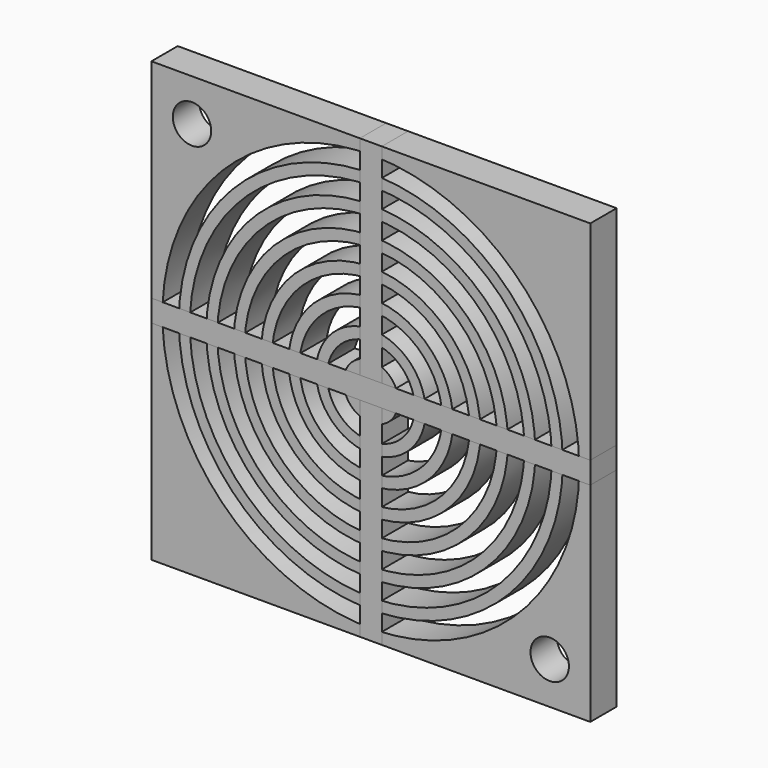
from build123d import *

# Parameters (mm, degrees)
F0_W      = 40
F0_H      = 40
F0_R      = 19
F1_DEPTH  = 3
F2_R      = 1.75
F3_DEPTH  = 5
F6_COUNT  = 2
F8_R      = 10
F8_R_2    = 9
F18_DEPTH = 3
F9_R      = 5
F9_R_2    = 4
F10_R     = 7.5
F10_R_2   = 6.5
F11_R     = 2.5
F11_R_2   = 1.5
F12_R     = 2.5
F13_R     = 12.5
F13_R_2   = 11.5
F14_R     = 15
F14_R_2   = 14
F15_R     = 17.5
F15_R_2   = 16.5
F16_W     = 2
F16_H     = 40
F17_W     = 40
F17_H     = 2


# Not quite as in the source:
# - a feature names something its author has since deleted; it is built from what else it names


with BuildPart() as f1:
    # F0 (on Front) → F1 (new body)
    with BuildSketch(Plane.XZ):
        Rectangle(F0_W, F0_H)
        Circle(F0_R, mode=Mode.SUBTRACT)
    extrude(amount=F1_DEPTH)


with BuildPart() as f3:
    # F2 (on face) → F3 (new body)
    with BuildSketch(Plane(origin=(0, 0, 0), x_dir=(-1, 0, 0), z_dir=(0, 1, 0))):
        with Locations((16.3023483751, 16.1759720192)):
            Circle(F2_R)
    extrude(amount=-F3_DEPTH)


with BuildPart() as f6_1:
    # F6: instance of F3
    add(f3.part.rotate(Axis((0, -5.2183736116, 0), (0, -1, 0)), 1 * 360 / F6_COUNT))


with BuildPart() as f1_1:
    add(f1.part)

    # F7: cut F6_1, F3
    add(f6_1.part, mode=Mode.SUBTRACT)
    add(f3.part, mode=Mode.SUBTRACT)


with BuildPart() as f18:
    # F8 (on face) → F18 (new body)
    with BuildSketch(Plane.XZ.offset(3)):
        Circle(F8_R)
        Circle(F8_R_2, mode=Mode.SUBTRACT)
    extrude(amount=-F18_DEPTH)


with BuildPart() as f18b:
    # F9 (on face) → F18, piece 2 (new body)
    with BuildSketch(Plane.XZ.offset(3)):
        Circle(F9_R)
        Circle(F9_R_2, mode=Mode.SUBTRACT)
    extrude(amount=-F18_DEPTH)


with BuildPart() as f18c:
    # F10 (on face) → F18, piece 3 (new body)
    with BuildSketch(Plane.XZ.offset(3)):
        Circle(F10_R)
        Circle(F10_R_2, mode=Mode.SUBTRACT)
    extrude(amount=-F18_DEPTH)


with BuildPart() as f18d:
    # F11 (on face) → F18, piece 4 (new body)
    with BuildSketch(Plane.XZ.offset(3)):
        Circle(F11_R)
        Circle(F11_R_2, mode=Mode.SUBTRACT)
    extrude(amount=-F18_DEPTH)


with BuildPart() as f18e:
    # F12 (on face) → F18, piece 5 (new body)
    with BuildSketch(Plane.XZ.offset(3)):
        Circle(F12_R)
    extrude(amount=-F18_DEPTH)


with BuildPart() as f18f:
    # F13 (on face) → F18, piece 6 (new body)
    with BuildSketch(Plane.XZ.offset(3)):
        Circle(F13_R)
        Circle(F13_R_2, mode=Mode.SUBTRACT)
    extrude(amount=-F18_DEPTH)


with BuildPart() as f18g:
    # F14 (on face) → F18, piece 7 (new body)
    with BuildSketch(Plane.XZ.offset(3)):
        Circle(F14_R)
        Circle(F14_R_2, mode=Mode.SUBTRACT)
    extrude(amount=-F18_DEPTH)


with BuildPart() as f18h:
    # F15 (on face) → F18, piece 8 (new body)
    with BuildSketch(Plane.XZ.offset(3)):
        Circle(F15_R)
        Circle(F15_R_2, mode=Mode.SUBTRACT)
    extrude(amount=-F18_DEPTH)


with BuildPart() as f18i:
    # F16 (on face) → F18, piece 9 (new body)
    with BuildSketch(Plane.XZ.offset(3)):
        Rectangle(F16_W, F16_H)
    extrude(amount=-F18_DEPTH)


with BuildPart() as f18j:
    # F17 (on face) → F18, piece 10 (new body)
    with BuildSketch(Plane.XZ.offset(3)):
        Rectangle(F17_W, F17_H)
    extrude(amount=-F18_DEPTH)


solid = Compound([f1_1.part, f18.part, f18b.part, f18c.part, f18d.part, f18e.part, f18f.part, f18g.part, f18h.part, f18i.part, f18j.part])
